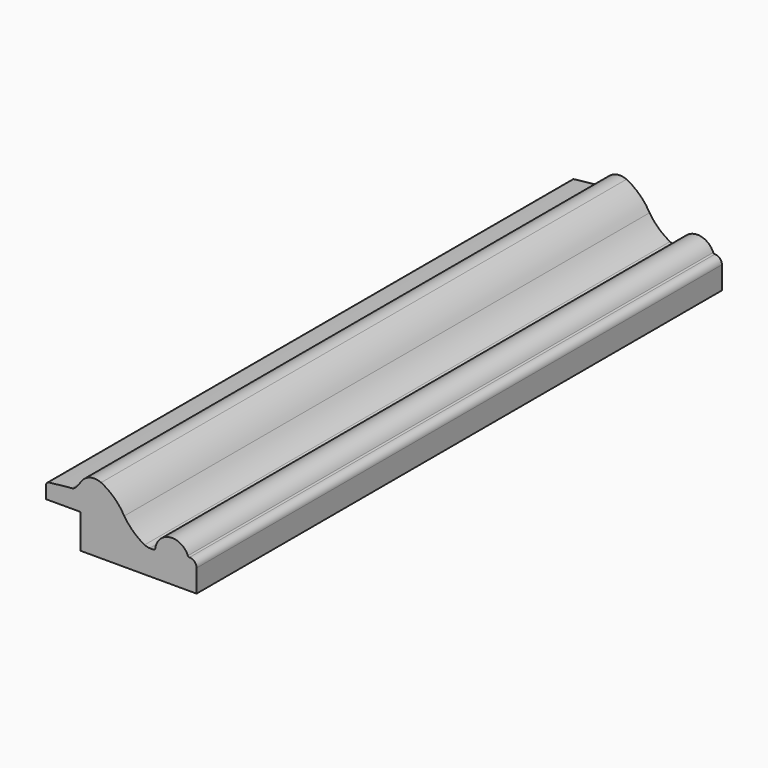
from build123d import *

# Parameters (mm, degrees)
F1_DEPTH = 152.4


# Not quite as in the source:
# - ends of sketch curves that miss each other by under 0.0002 mm in the source are joined


with BuildPart() as f1:
    # F0 (on Front) → F1 (new body)
    with BuildSketch(Plane.XZ):
        with BuildLine():
            Line((-9.4615, 0.028575), (-9.4615, -7.908925))
            Line((-9.4615, -7.908925), (17.4625, -7.908925))
            Line((17.4625, -7.908925), (17.4625, -2.65938))
            ThreePointArc((17.4625, -2.65938), (16.9760741715, -1.5035311682), (15.8095437434, -1.0433101682))
            ThreePointArc((15.8095437434, -1.0433101682), (15.5930919547, -0.9817228233), (15.4491526844, -0.8087322213))
            ThreePointArc((15.4491526844, -0.8087322213), (11.2653307166, 1.5970590296), (7.8607199392, -1.8235935338))
            ThreePointArc((7.8607199392, -1.8235935338), (7.736905149, -2.0587727487), (7.4894692803, -2.1557927219))
            Line((7.4894692803, -2.1557927219), (7.4829161901, -2.1558009151))
            Line((7.4829161901, -2.1558009151), (6.603492, -2.1559774))
            ThreePointArc((6.603492, -2.1559774), (5.9901232061, -2.0809037525), (5.413035163, -1.8599360759))
            ThreePointArc((5.413035163, -1.8599360759), (2.7666336142, 0.0131384296), (0.682874392, 2.4970459891))
            ThreePointArc((0.682874392, 2.4970459891), (-1.6202189431, 5.441919304), (-4.6831053409, 7.585571483))
            ThreePointArc((-4.6831053409, 7.585571483), (-7.435761648, 7.7094554069), (-9.5520790293, 5.9448968563))
            ThreePointArc((-9.5520790293, 5.9448968563), (-10.089729001, 5.2101835463), (-10.7216915696, 4.5548251488))
            ThreePointArc((-10.7216915696, 4.5548251488), (-11.0931160448, 4.3208677831), (-11.52199893, 4.2273251642))
            ThreePointArc((-11.52199893, 4.2273251642), (-14.1558174385, 3.9550500254), (-16.7874935974, 3.6627947922))
            ThreePointArc((-16.7874935974, 3.6627947922), (-17.2692415305, 3.4129116875), (-17.4625, 2.9057854))
            Line((-17.4625, 2.9057854), (-17.4625, 0.028575))
            Line((-17.4625, 0.028575), (-9.4615, 0.028575))
        make_face()
    extrude(amount=F1_DEPTH)


solid = f1.part
